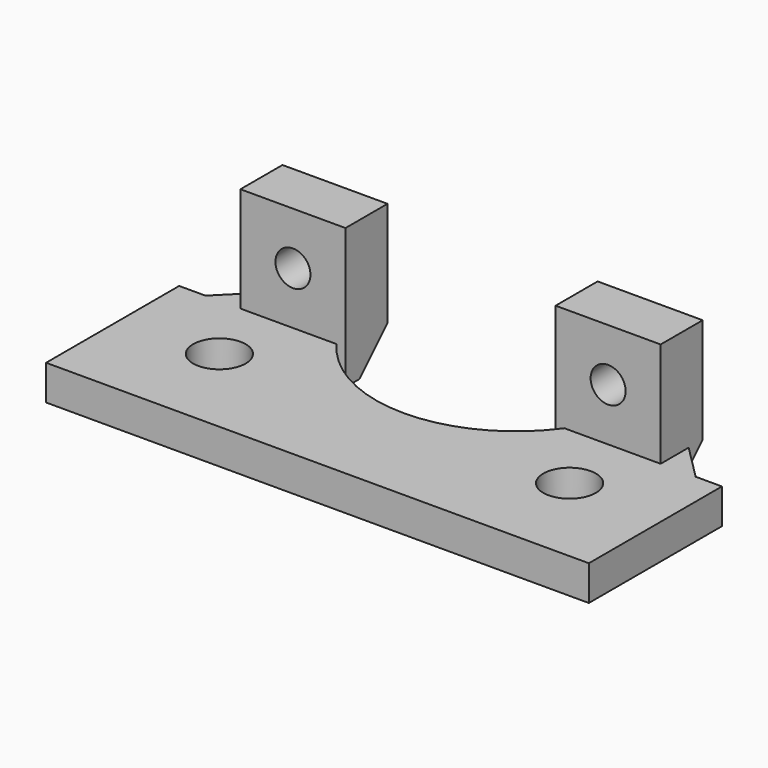
from build123d import *

# Parameters (mm, degrees)
F0_R     = 1.5
F1_DEPTH = 2
F2_W     = 6
F2_H     = 8
F2_R     = 1
F3_DEPTH = 3
F4_SIZE  = 2
F5_SIZE  = 2


with BuildPart() as f1:
    # F0 (on Top) → F1 (new body)
    with BuildSketch(Plane.XY):
        with BuildLine():
            Line((-6.5, 0), (-15.5, 0))
            Line((-15.5, 0), (-15.5, -9.5))
            Line((-15.5, -9.5), (15.5, -9.5))
            Line((15.5, -9.5), (15.5, 0))
            Line((15.5, 0), (6.5, 0))
            ThreePointArc((6.5, 0), (0, -3.3363104735), (-6.5, 0))
        make_face()
        with Locations((-10, -4)):
            Circle(F0_R, mode=Mode.SUBTRACT)
        with Locations((10, -4)):
            Circle(F0_R, mode=Mode.SUBTRACT)
    extrude(amount=F1_DEPTH)

    # F2 (on Front) → F3 (join)
    with BuildSketch(Plane.XZ):
        with Locations((-9, 4)):
            Rectangle(F2_W, F2_H)
        with Locations((-9, 5)):
            Circle(F2_R, mode=Mode.SUBTRACT)
        with Locations((9, 4)):
            Rectangle(F2_W, F2_H)
        with Locations((9, 5)):
            Circle(F2_R, mode=Mode.SUBTRACT)
    extrude(amount=-F3_DEPTH)

    # F4
    f4_edges = [f1.edges().sort_by_distance(p)[0] for p in [
        (9, 3, 0),
        (-9, 3, 0),
    ]]
    chamfer(f4_edges, length=F4_SIZE)

    # F5
    f5_edges = [f1.edges().sort_by_distance(p)[0] for p in [
        (-12, 0, 1),
        (12, 0, 1),
    ]]
    chamfer(f5_edges, length=F5_SIZE)


solid = f1.part
